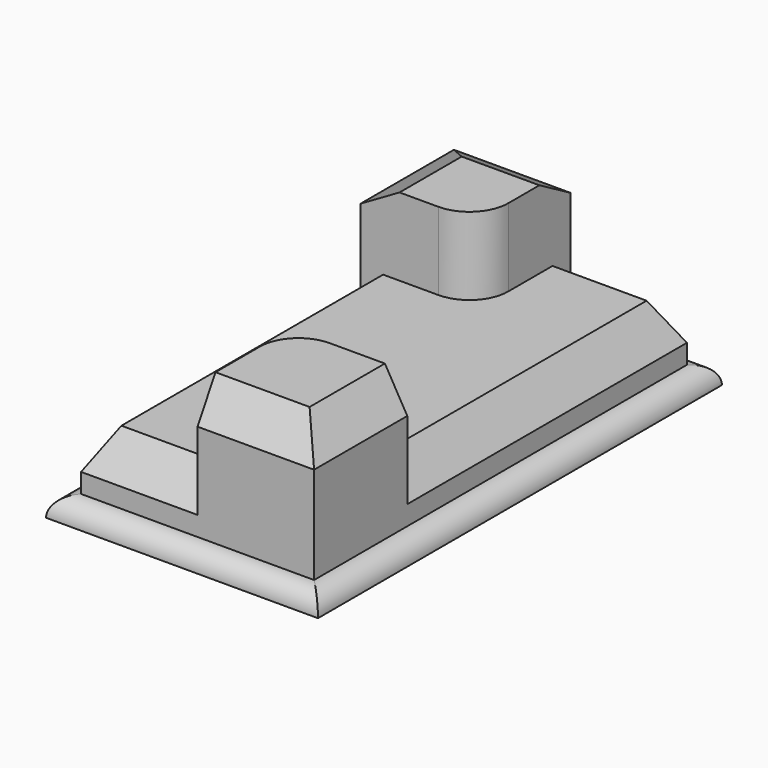
from build123d import *

# Parameters (mm, degrees)
F0_W        = 88.9
F0_H        = 165.1
F1_DEPTH    = 6.35
F2_DEPTH    = 25.4
F3_DEPTH    = 50.8
F4_R        = 6.34999
F5_C1_SIZE2 = 7.3323484187
F5_C1_SIZE  = 12.7
F5_C2_SIZE2 = 12.7
F5_C2_SIZE  = 7.3323484187
F5_C3_SIZE2 = 7.3323484187
F5_C3_SIZE  = 12.7
F5_C4_SIZE2 = 7.3323484187
F5_C4_SIZE  = 12.7
F5_C5_SIZE2 = 7.3323484187
F5_C5_SIZE  = 12.7
F5_C6_SIZE2 = 7.3323484187
F5_C6_SIZE  = 12.7
F5_C7_SIZE2 = 12.7
F5_C7_SIZE  = 7.3323484187
F5_C8_SIZE2 = 7.3323484187
F5_C8_SIZE  = 12.7


# Not quite as in the source:
# - a fillet or chamfer is up to 0.001 mm smaller than in the source, because OpenCascade refuses the exact size


with BuildPart() as f1:
    # F0 (on Top) → F1 (new body)
    with BuildSketch(Plane.XY):
        Rectangle(F0_W, F0_H)
        Polygon((0, 76.2), (38.1, 76.2), (38.1, -38.1), (38.1, -76.2), (0, -76.2), (-38.1, -76.2), (-38.1, 38.1), (-38.1, 76.2), align=None, mode=Mode.SUBTRACT)
    extrude(amount=F1_DEPTH)

    # F0 (on Top) → F2 (join)
    with BuildSketch(Plane.XY):
        with BuildLine():
            Line((38.1, -38.1), (38.1, 76.2))
            Line((38.1, 76.2), (0, 76.2))
            Line((0, 76.2), (0, 50.8))
            ThreePointArc((0, 50.8), (-3.7197438789, 41.8197438789), (-12.7, 38.1))
            Line((-12.7, 38.1), (-38.1, 38.1))
            Line((-38.1, 38.1), (-38.1, -76.2))
            Line((-38.1, -76.2), (0, -76.2))
            Line((0, -76.2), (0, -50.8))
            ThreePointArc((0, -50.8), (3.7197438789, -41.8197438789), (12.7, -38.1))
            Line((12.7, -38.1), (38.1, -38.1))
        make_face()
    extrude(amount=F2_DEPTH)

    # F0 (on Top) → F3 (join)
    with BuildSketch(Plane.XY):
        with BuildLine():
            Line((0, 50.8), (0, 76.2))
            Line((0, 76.2), (-38.1, 76.2))
            Line((-38.1, 76.2), (-38.1, 38.1))
            Line((-38.1, 38.1), (-12.7, 38.1))
            ThreePointArc((-12.7, 38.1), (-3.7197438789, 41.8197438789), (0, 50.8))
        make_face()
        with BuildLine():
            Line((38.1, -76.2), (38.1, -38.1))
            Line((38.1, -38.1), (12.7, -38.1))
            ThreePointArc((12.7, -38.1), (3.7197438789, -41.8197438789), (0, -50.8))
            Line((0, -50.8), (0, -76.2))
            Line((0, -76.2), (38.1, -76.2))
        make_face()
    extrude(amount=F3_DEPTH)

    # F4 (radius 6.35 in the source; OpenCascade refuses exactly that, so slightly less here)
    f4_edges = [f1.edges().sort_by_distance(p)[0] for p in [
        (44.45, 0, 6.35),
        (0, -82.55, 6.35),
        (-44.45, 0, 6.35),
        (0, 82.55, 6.35),
    ]]
    fillet(f4_edges, radius=F4_R)

    # F5: chamfer of 12.7 x 7.3323484187 on 8 edges, made by hand

    # F5_c1
    f5_c1_edges = [f1.edges().sort_by_distance(p)[0] for p in [
        (19.05, 76.2, 25.4),
    ]]
    f5_c1_side = f1.faces().sort_by_distance((19.05, 76.2, 25.2533530316))[0]
    chamfer(f5_c1_edges, length=F5_C1_SIZE, length2=F5_C1_SIZE2, reference=f5_c1_side)

    # F5_c2
    f5_c2_edges = [f1.edges().sort_by_distance(p)[0] for p in [
        (-19.05, 76.2, 50.8),
    ]]
    f5_c2_side = f1.faces().sort_by_distance((-19.05, 76.2, 50.6533530316))[0]
    chamfer(f5_c2_edges, length=F5_C2_SIZE, length2=F5_C2_SIZE2, reference=f5_c2_side)

    # F5_c3
    f5_c3_edges = [f1.edges().sort_by_distance(p)[0] for p in [
        (38.1, -57.15, 50.8),
    ]]
    f5_c3_side = f1.faces().sort_by_distance((38.1, -57.15, 50.6533530316))[0]
    chamfer(f5_c3_edges, length=F5_C3_SIZE, length2=F5_C3_SIZE2, reference=f5_c3_side)

    # F5_c4
    f5_c4_edges = [f1.edges().sort_by_distance(p)[0] for p in [
        (38.1, 15.3838257906, 25.4),
    ]]
    f5_c4_side = f1.faces().sort_by_distance((38.1, 15.3838257906, 25.2533530316))[0]
    chamfer(f5_c4_edges, length=F5_C4_SIZE, length2=F5_C4_SIZE2, reference=f5_c4_side)

    # F5_c5
    f5_c5_edges = [f1.edges().sort_by_distance(p)[0] for p in [
        (-19.05, -76.2, 25.4),
    ]]
    f5_c5_side = f1.faces().sort_by_distance((-19.05, -76.2, 25.2533530316))[0]
    chamfer(f5_c5_edges, length=F5_C5_SIZE, length2=F5_C5_SIZE2, reference=f5_c5_side)

    # F5_c6
    f5_c6_edges = [f1.edges().sort_by_distance(p)[0] for p in [
        (15.3838257906, -76.2, 50.8),
    ]]
    f5_c6_side = f1.faces().sort_by_distance((15.3838257906, -76.2, 50.6533530316))[0]
    chamfer(f5_c6_edges, length=F5_C6_SIZE, length2=F5_C6_SIZE2, reference=f5_c6_side)

    # F5_c7
    f5_c7_edges = [f1.edges().sort_by_distance(p)[0] for p in [
        (-38.1, 50.8, 50.8),
    ]]
    f5_c7_side = f1.faces().sort_by_distance((-38.1, 50.8, 50.6533530316))[0]
    chamfer(f5_c7_edges, length=F5_C7_SIZE, length2=F5_C7_SIZE2, reference=f5_c7_side)

    # F5_c8
    f5_c8_edges = [f1.edges().sort_by_distance(p)[0] for p in [
        (-38.1, -15.3838257906, 25.4),
    ]]
    f5_c8_side = f1.faces().sort_by_distance((-38.1, -15.3838257906, 25.2533530316))[0]
    chamfer(f5_c8_edges, length=F5_C8_SIZE, length2=F5_C8_SIZE2, reference=f5_c8_side)


solid = f1.part
